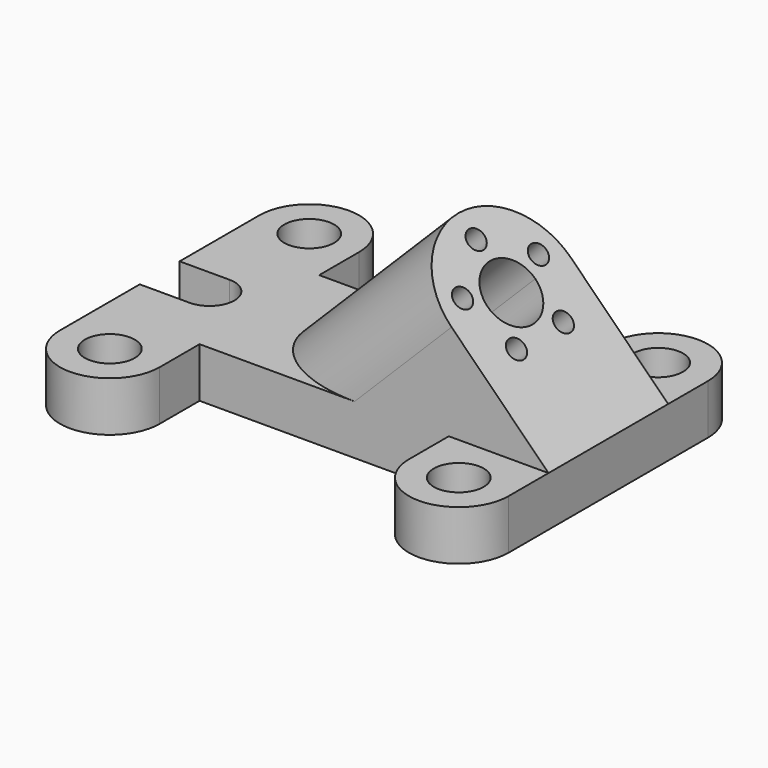
from build123d import *

# Parameters (mm, degrees)
F0_R             = 6.35
F1_DEPTH         = 12.7
F3_DEPTH         = 38.1
F7_DEPTH         = 89.8035612107
F8_R             = 2.54
F9_DEPTH         = 6.35
F9_COPIES_COUNT  = 2
F9_COPIES_PITCH  = 14.929745
F9_COPIES1_COUNT = 2
F9_COPIES1_PITCH = 14.929745
F9_COPIES2_COUNT = 2
F9_COPIES2_PITCH = 24.156836
F9_COPIES3_COUNT = 2
F9_COPIES3_PITCH = 24.156836


# Not quite as in the source:
# - a pattern or mirror of a feature is missing from the dataset's text; its kind, count and spacing are read off the source's solid


with BuildPart() as f1:
    # F0 (on Top) → F1 (new body)
    with BuildSketch(Plane.XY):
        with BuildLine():
            Line((12.7, 50.8), (12.7, 63.5))
            ThreePointArc((12.7, 63.5), (0, 76.2), (-12.7, 63.5))
            Line((-12.7, 63.5), (-12.7, 38.1))
            Line((-12.7, 38.1), (0, 38.1))
            ThreePointArc((0, 38.1), (6.35, 31.75), (0, 25.4))
            Line((0, 25.4), (-12.7, 25.4))
            Line((-12.7, 25.4), (-12.7, 0))
            ThreePointArc((-12.7, 0), (0, -12.7), (12.7, 0))
            Line((12.7, 0), (12.7, 12.7))
            Line((12.7, 12.7), (76.2, 12.7))
            Line((76.2, 12.7), (76.2, 0))
            ThreePointArc((76.2, 0), (88.9, -12.7), (101.6, 0))
            Line((101.6, 0), (101.6, 63.5))
            ThreePointArc((101.6, 63.5), (88.9, 76.2), (76.2, 63.5))
            Line((76.2, 63.5), (76.2, 50.8))
            Line((76.2, 50.8), (12.7, 50.8))
        make_face()
        Circle(F0_R, mode=Mode.SUBTRACT)
        with Locations((88.9, 0)):
            Circle(F0_R, mode=Mode.SUBTRACT)
        with Locations((0, 63.5)):
            Circle(F0_R, mode=Mode.SUBTRACT)
        with Locations((88.9, 63.5)):
            Circle(F0_R, mode=Mode.SUBTRACT)
    extrude(amount=F1_DEPTH)

    # F2 (on face) → F3 (join)
    with BuildSketch(Plane.XZ.offset(-12.7)):
        Polygon((76.2, 12.7), (101.6, 12.7), (76.9042956671, 37.3957043329), (52.2085913341, 12.7), align=None)
    extrude(amount=-F3_DEPTH)

    # F4 (on face) → F5 (join, up to the next surface of F1)
    with BuildSketch(Plane(origin=(57.15, 0, 57.15), x_dir=(0.7071067812, 0, -0.7071067812), z_dir=(0.7071067812, 0, 0.7071067812))):
        with BuildLine():
            ThreePointArc((27.9367928475, 24.13), (20.3167928475, 31.75), (27.9367928475, 39.37))
            Line((27.9367928475, 39.37), (27.9367928475, 50.8))
            ThreePointArc((27.9367928475, 50.8), (8.8867928475, 31.75), (27.9367928475, 12.7))
            Line((27.9367928475, 12.7), (27.9367928475, 24.13))
        make_face()
    extrude(until=Until.NEXT, dir=(-0.7071067812, 0, -0.7071067812))

    # F6 (on face) → F7 (cut, through all)
    with BuildSketch(Plane(origin=(57.15, 0, 57.15), x_dir=(0.7071067812, 0, -0.7071067812), z_dir=(0.7071067812, 0, 0.7071067812))):
        with BuildLine():
            ThreePointArc((27.9367928475, 24.13), (33.3249465201, 26.3618463274), (35.5567928475, 31.75))
            ThreePointArc((35.5567928475, 31.75), (33.3249465201, 37.1381536726), (27.9367928475, 39.37))
            Line((27.9367928475, 39.37), (27.9367928475, 24.13))
        make_face()
        with BuildLine():
            Line((27.9367928475, 24.13), (27.9367928475, 39.37))
            ThreePointArc((27.9367928475, 39.37), (20.3167928475, 31.75), (27.9367928475, 24.13))
        make_face()
    extrude(amount=-F7_DEPTH, mode=Mode.SUBTRACT)

    # F8 (on face) → F9 (cut)
    with BuildSketch(Plane(origin=(57.15, 0, 57.15), x_dir=(0.7071067812, 0, -0.7071067812), z_dir=(0.7071067812, 0, 0.7071067812))):
        with Locations((15.2367928475, 31.75)):
            Circle(F8_R)
    f9 = extrude(amount=-F9_DEPTH, mode=Mode.SUBTRACT)

    # F9_copies: F9 ×2
    with Locations(*[Vector(0.4156269378, 0.8090169944, -0.4156269378) * (i * F9_COPIES_PITCH) for i in range(1, F9_COPIES_COUNT)]):
        add(f9, mode=Mode.SUBTRACT)

    # F9_copies1: F9 ×2
    with Locations(*[Vector(0.4156269378, -0.8090169944, -0.4156269378) * (i * F9_COPIES1_PITCH) for i in range(1, F9_COPIES1_COUNT)]):
        add(f9, mode=Mode.SUBTRACT)

    # F9_copies2: F9 ×2
    with Locations(*[Vector(0.672498512, -0.3090169944, -0.672498512) * (i * F9_COPIES2_PITCH) for i in range(1, F9_COPIES2_COUNT)]):
        add(f9, mode=Mode.SUBTRACT)

    # F9_copies3: F9 ×2
    with Locations(*[Vector(0.672498512, 0.3090169944, -0.672498512) * (i * F9_COPIES3_PITCH) for i in range(1, F9_COPIES3_COUNT)]):
        add(f9, mode=Mode.SUBTRACT)


solid = f1.part
